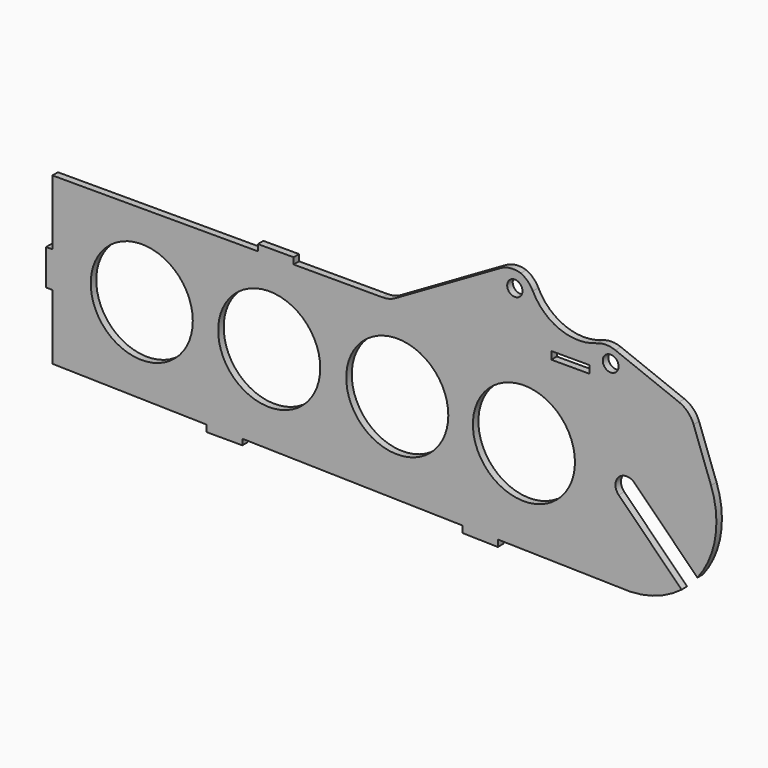
from build123d import *

# Parameters (mm, degrees)
F0_R     = 25.4
F0_W     = 19.05
F0_H     = 3.81
F0_R_2   = 3.81
F0_R_3   = 3.937
F1_DEPTH = 3.429


# Not quite as in the source:
# - ends of sketch curves that miss each other by under 0.0002 mm in the source are joined


with BuildPart() as f1:
    # F0 (on Front) → F1 (new body)
    with BuildSketch(Plane.XZ):
        with BuildLine():
            Line((122.9326218, 166.8279366), (126.1076218, 166.8279366))
            Line((126.1076218, 166.8279366), (126.1076218, 134.4429366))
            Line((126.1076218, 134.4429366), (202.8156218, 132.7586372))
            Line((202.8156218, 132.7586372), (202.8156218, 129.4566372))
            Line((202.8156218, 129.4566372), (220.5956218, 129.4566372))
            Line((220.5956218, 129.4566372), (220.5956218, 132.3682392))
            Line((220.5956218, 132.3682392), (330.0696218, 129.9644848))
            Line((330.0696218, 129.9644848), (330.0696218, 126.6616974))
            Line((330.0696218, 126.6616974), (347.7771302, 126.2728742))
            Line((347.7771302, 126.2728742), (347.8496218, 129.5740868))
            Line((347.8496218, 129.5740868), (413.8162158, 128.1256518))
            ThreePointArc((413.8162158, 128.1256518), (427.2355191442, 130.7449674015), (439.2238892088, 137.3189752107))
            Line((439.2238892088, 137.3189752107), (407.9287752, 168.61409))
            ThreePointArc((407.9287752, 168.61409), (407.928759747, 176.471798653), (415.786483853, 176.471798653))
            Line((415.786483853, 176.471798653), (447.1136092, 145.1446932))
            ThreePointArc((447.1136092, 145.1446932), (456.0111791953, 165.5693177048), (453.8809524214, 187.7457494791))
            Line((453.8809524214, 187.7457494791), (445.1949186, 211.6104734))
            ThreePointArc((445.1949186, 211.6104734), (442.3538053066, 216.1328975514), (437.9046056469, 219.0873571921))
            Line((437.9046056469, 219.0873571921), (406.246711, 231.5244036))
            ThreePointArc((406.246711, 231.5244036), (401.6620386638, 232.4037156495), (397.069381607, 231.5671130188))
            ThreePointArc((397.069381607, 231.5671130188), (378.7147395647, 231.6525545857), (365.2100276158, 244.0832755023))
            ThreePointArc((365.2100276158, 244.0832755023), (362.7212006534, 247.5307318984), (359.2339287197, 249.9634606203))
            ThreePointArc((359.2339287197, 249.9634606203), (354.0189561213, 250.4862087964), (349.0369734787, 248.858627921))
            Line((349.0369734787, 248.858627921), (296.7910244, 218.6944318))
            ThreePointArc((296.7910244, 218.6944318), (293.728030578, 217.4256797597), (290.4410244, 216.9929366))
            Line((290.4410244, 216.9929366), (246.1226218, 216.9929366))
            Line((246.1226218, 216.9929366), (246.1226218, 220.1679366))
            Line((246.1226218, 220.1679366), (228.3426218, 220.1679366))
            Line((228.3426218, 220.1679366), (228.3426218, 216.9929366))
            Line((228.3426218, 216.9929366), (126.1076218, 216.9929366))
            Line((126.1076218, 216.9929366), (126.1076218, 184.6079366))
            Line((126.1076218, 184.6079366), (122.9326218, 184.6079366))
            Line((122.9326218, 184.6079366), (122.9326218, 166.8279366))
        make_face()
        with Locations((170.5510686, 175.9319824)):
            Circle(F0_R, mode=Mode.SUBTRACT)
        with Locations((233.9839364, 175.9319824)):
            Circle(F0_R, mode=Mode.SUBTRACT)
        with Locations((297.721782, 175.9319824)):
            Circle(F0_R, mode=Mode.SUBTRACT)
        with Locations((360.7561746, 175.9319824)):
            Circle(F0_R, mode=Mode.SUBTRACT)
        with Locations((383.9176218, 218.8979366)):
            Rectangle(F0_W, F0_H, mode=Mode.SUBTRACT)
        with Locations((356.2316218, 242.3929366)):
            Circle(F0_R_2, mode=Mode.SUBTRACT)
        with Locations((403.935946, 224.9304366)):
            Circle(F0_R_3, mode=Mode.SUBTRACT)
    extrude(amount=F1_DEPTH)


solid = f1.part
